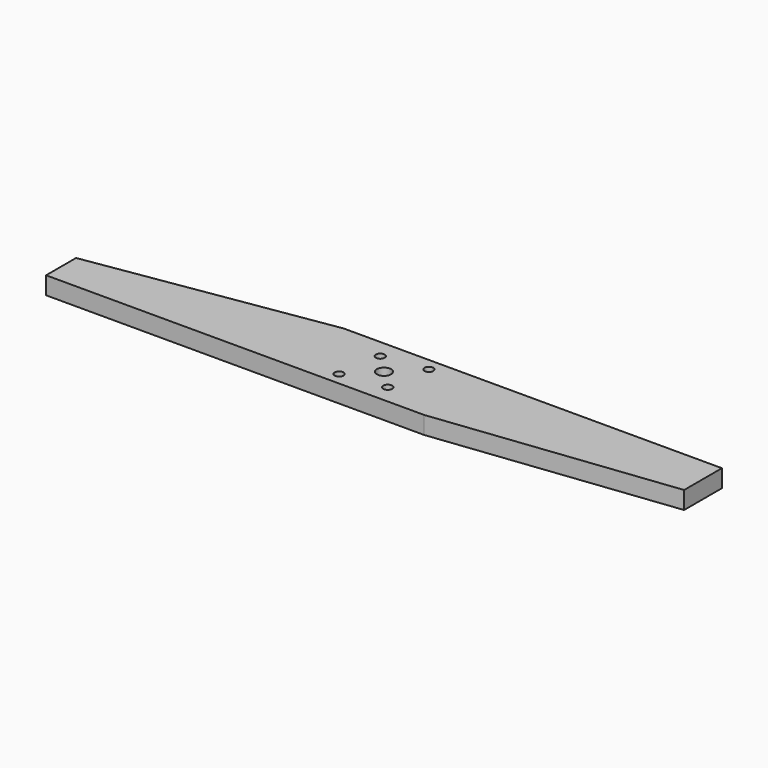
from build123d import *

# Parameters (mm, degrees)
F0_R     = 1
F0_R_2   = 1.6
F1_DEPTH = 4


# Not quite as in the source:
# - a feature names something its author has since deleted; it is built from what else it names


with BuildPart() as f1:
    # F0 (on Top) → F1 (new body)
    with BuildSketch(Plane.XY):
        Polygon((-69.85, 0), (-69.85, -8.5), (15.9242544323, -8.5), (69.85, -2.218887916), (69.85, 8.5), (-15.9242544323, 8.5), align=None)
        with Locations((-5.6605379174, -5.6497372861)):
            Circle(F0_R, mode=Mode.SUBTRACT)
        with Locations((4.2389570192, -4.2355237237)):
            Circle(F0_R, mode=Mode.SUBTRACT)
        with Locations((-4.2463243551, 4.2497576505)):
            Circle(F0_R, mode=Mode.SUBTRACT)
        Circle(F0_R_2, mode=Mode.SUBTRACT)
        with Locations((5.6531705815, 5.6639712129)):
            Circle(F0_R, mode=Mode.SUBTRACT)
    extrude(amount=F1_DEPTH)


solid = f1.part
